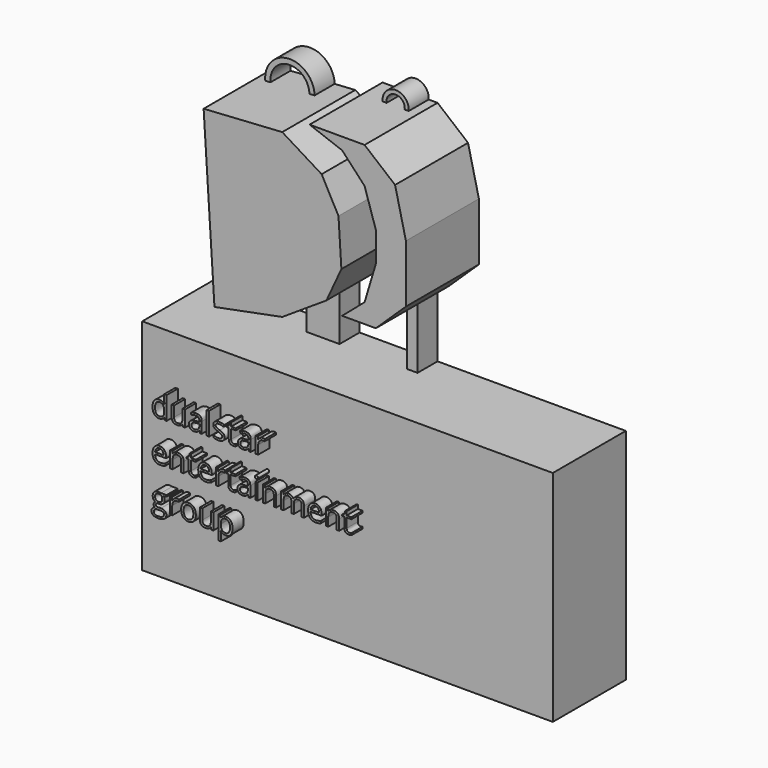
from build123d import *

# Parameters (mm, degrees)
F1_DEPTH     = 15.748
F0_W         = 70.8931386471
F0_H         = 37.8373926505
F2_TEXT_SIZE = 5.1612517481
F3_DEPTH     = 18.161
F4_W         = 5.7103279978
F4_H         = 15.9504665062
F5_DEPTH     = 4.318
F4_W_2       = 1.8455855316
F4_H_2       = 16.3409588858
F4_R         = 4.2739346802
F4_R_2       = 3.3713500943
F4_R_3       = 2.2647028386
F4_R_4       = 1.5797726873


# Not quite as in the source:
# - Text() gives the source's letters only with a copy of the font that has no kerning and outlines rounded to 1/6400 em; it was checked with that copy


with BuildPart() as f1:
    # F0 (on Front) → F1 (new body)
    with BuildSketch(Plane.XZ):
        Polygon((-27.7909543365, 47.919690609), (-25.9198751301, 18.3982104063), (-14.213553326, 20.6850860268), (-6.5853861161, 25.6746318191), (-4.0052034121, 31.2801078803), (-4.5064068399, 39.1879864037), (-7.4169770814, 44.5933267474), (-14.213553326, 48.7802298683), align=None)
    extrude(amount=F1_DEPTH)


with BuildPart() as f1b:
    # F0 (on Front) → F1, piece 2 (new body)
    with BuildSketch(Plane.XZ):
        Polygon((0, 51.4539554715), (-9.4959540293, 51.4539554715), (-3.8827138487, 49.3749789894), (0, 45.2170222998), (1.9384231418, 39.1879864037), (1.9384231418, 33.9905433357), (0, 27.5457128882), (-3.8827138487, 24.219347164), (1.9384231418, 24.219347164), (7.1358666755, 29.208894819), (7.1358666755, 33.9905433357), (7.1358666755, 39.1879864037), (5.2647874691, 47.0881015062), align=None)
    extrude(amount=F1_DEPTH)


with BuildPart() as f1c:
    # F0 (on Front) → F1, piece 3 (new body)
    with BuildSketch(Plane.XZ):
        with Locations((-2.9471740127, -6.7574181594)):
            Rectangle(F0_W, F0_H)
    extrude(amount=F1_DEPTH)

    # F2 (on Front) → F3 (join)
    with BuildSketch(Plane.XZ):
        with Locations((-34.9666741481, 0)):
            Text('dualstar', F2_TEXT_SIZE, font='Open Sans', text_align=(TextAlign.LEFT, TextAlign.BOTTOM))
        with Locations((-34.9666741481, -7.0193023775)):
            Text('entertainment', F2_TEXT_SIZE, font='Open Sans', text_align=(TextAlign.LEFT, TextAlign.BOTTOM))
        with Locations((-34.9666741481, -14.038604755)):
            Text('group', F2_TEXT_SIZE, font='Open Sans', text_align=(TextAlign.LEFT, TextAlign.BOTTOM))
    extrude(amount=F3_DEPTH)


with BuildPart() as f5:
    # F4 (on Front) → F5 (new body)
    with BuildSketch(Plane.XZ):
        with Locations((-16.3183091208, 17.7191295661)):
            Rectangle(F4_W, F4_H)
    extrude(amount=F5_DEPTH)


with BuildPart() as f5b:
    # F4 (on Front) → F5, piece 2 (new body)
    with BuildSketch(Plane.XZ):
        with Locations((-0.9227927658, 17.9143757559)):
            Rectangle(F4_W_2, F4_H_2)
    extrude(amount=F5_DEPTH)


with BuildPart() as f5c:
    # F4 (on Front) → F5, piece 3 (new body)
    with BuildSketch(Plane.XZ):
        with Locations((-22.0366213471, 48.4189651906)):
            Circle(F4_R)
        with Locations((-22.0366213471, 48.4189651906)):
            Circle(F4_R_2, mode=Mode.SUBTRACT)
    extrude(amount=F5_DEPTH)


with BuildPart() as f5d:
    # F4 (on Front) → F5, piece 4 (new body)
    with BuildSketch(Plane.XZ):
        with Locations((-3.7851158995, 51.659271121)):
            Circle(F4_R_3)
        with Locations((-3.7851158995, 51.659271121)):
            Circle(F4_R_4, mode=Mode.SUBTRACT)
    extrude(amount=F5_DEPTH)


solid = Compound([f1.part, f1b.part, f1c.part, f5.part, f5b.part, f5c.part, f5d.part])
